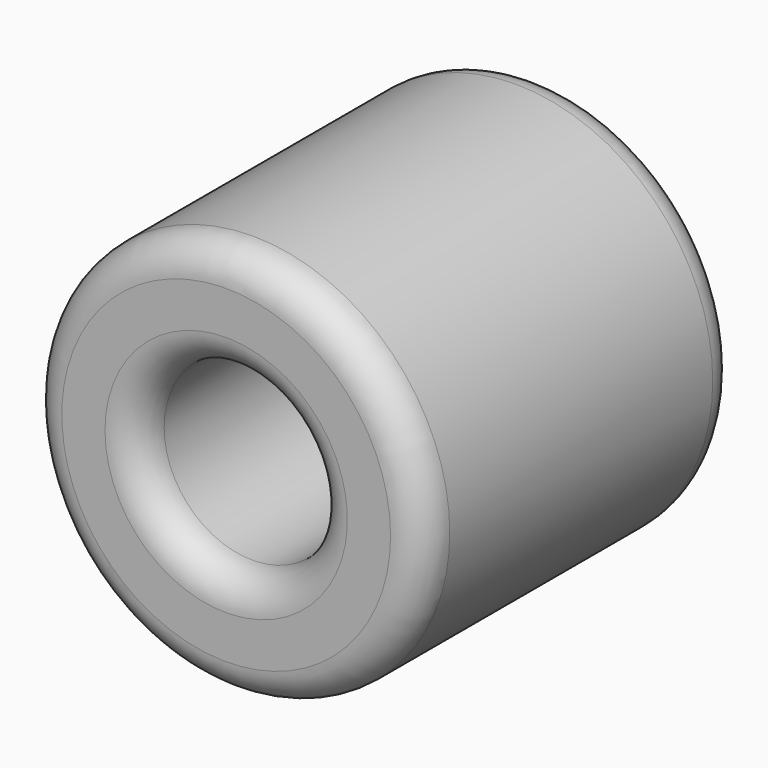
from build123d import *

# Parameters (mm, degrees)
F0_R     = 38.1
F1_DEPTH = 38.1
F3_D     = 34.12998
F4_R     = 6.35


with BuildPart() as f1:
    # F0 (on Front) → F1 (new body, symmetric)
    with BuildSketch(Plane.XZ):
        Circle(F0_R)
    extrude(amount=F1_DEPTH, both=True)

    # F3 (through all)
    with Locations(Plane.XZ.offset(38.1)):
        with Locations((0, 0)):
            Hole(F3_D / 2)

    # F4
    f4_edges = [f1.edges().sort_by_distance(p)[0] for p in [
        (-38.1, -38.1, 0),
        (-38.1, 38.1, 0),
        (-17.06499, 38.1, 0),
        (-17.06499, -38.1, 0),
    ]]
    fillet(f4_edges, radius=F4_R)


solid = f1.part
